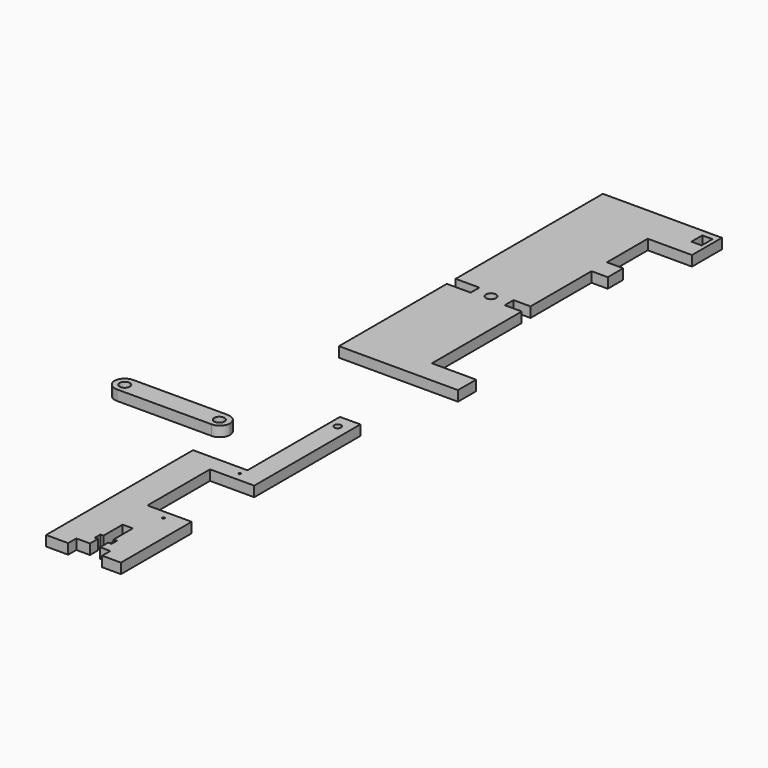
from build123d import *

# Parameters (mm, degrees)
F0_W        = 34
F0_H        = 6
F1_DEPTH    = 3
F2_T1_DEPTH = 18.5
F3_T1_DEPTH = 18.5
F4_R        = 1.5
F5_DEPTH    = 25.8
F6_W        = 35
F6_H        = 97
F7_DEPTH    = 3
F9_DEPTH    = 65
F10_W       = 13
F10_H       = 58.6508959532
F11_DEPTH   = 25
F12_W       = 5
F12_H       = 3.23662889
F12_W_2     = 7
F12_H_2     = 3.2004637718
F13_DEPTH   = 35.3
F14_R       = 1.5
F15_DEPTH   = 25
F16_W       = 8.2240308821
F16_H       = 5.6709373705
F16_W_2     = 3
F16_H_2     = 4
F17_DEPTH   = 25
F18_W       = 22
F18_H       = 88
F19_DEPTH   = 3
F20_W       = 16
F20_H       = 34
F21_DEPTH   = 14.5
F22_W       = 13
F22_H       = 23
F23_DEPTH   = 25
F24_W       = 10
F24_H       = 3
F25_DEPTH   = 25
F26_W       = 3
F26_H       = 12
F27_DEPTH   = 25
F29_DEPTH   = 25
F30_R       = 1
F30_R_2     = 0.35
F31_DEPTH   = 25


# Not quite as in the source:
# - a fillet or chamfer that OpenCascade refuses, or shapes differently, is made with other operations: its cross-section is extruded or revolved along the edge and cut away or added


with BuildPart() as f1:
    # F0 (on Top) → F1 (new body)
    with BuildSketch(Plane.XY):
        with Locations((-28.7276850939, -1.7022728249)):
            Rectangle(F0_W, F0_H)
    extrude(amount=F1_DEPTH)

    # F2: fillet of radius 3.1 on 2 edges, made by hand

    # F2_s2 → F2_t1 (cut)
    with BuildSketch(Plane.XY.offset(-7.75)):
        with BuildLine():
            ThreePointArc((-14.8276850939, -4.7022728249), (-12.6356540722, -3.7943038466), (-11.7276850939, -1.6022728249))
            Line((-11.7276850939, -1.6022728249), (-11.7276850939, -4.7022728249))
            Line((-11.7276850939, -4.7022728249), (-14.8276850939, -4.7022728249))
        make_face()
        with BuildLine():
            ThreePointArc((-14.8276850939, 1.2977271751), (-12.6356540722, 0.3897581967), (-11.7276850939, -1.8022728249))
            Line((-11.7276850939, -1.8022728249), (-11.7276850939, 1.2977271751))
            Line((-11.7276850939, 1.2977271751), (-14.8276850939, 1.2977271751))
        make_face()
    extrude(amount=F2_T1_DEPTH, mode=Mode.SUBTRACT)

    # F3: fillet of radius 3.1 on 2 edges, made by hand

    # F3_s2 → F3_t1 (cut)
    with BuildSketch(Plane.XY.offset(-7.75)):
        with BuildLine():
            ThreePointArc((-45.7276850939, -1.6022728249), (-44.8197161156, -3.7943038466), (-42.6276850939, -4.7022728249))
            Line((-42.6276850939, -4.7022728249), (-45.7276850939, -4.7022728249))
            Line((-45.7276850939, -4.7022728249), (-45.7276850939, -1.6022728249))
        make_face()
        with BuildLine():
            ThreePointArc((-42.6276850939, 1.2977271751), (-44.8197161156, 0.3897581967), (-45.7276850939, -1.8022728249))
            Line((-45.7276850939, -1.8022728249), (-45.7276850939, 1.2977271751))
            Line((-45.7276850939, 1.2977271751), (-42.6276850939, 1.2977271751))
        make_face()
    extrude(amount=F3_T1_DEPTH, mode=Mode.SUBTRACT)

    # F4 (on face) → F5 (cut)
    with BuildSketch(Plane(origin=(0, 0, 0), x_dir=(1, 0, 0), z_dir=(0, 0, -1))):
        with Locations((-42.6276850939, 1.8022728249)):
            Circle(F4_R)
        with Locations((-14.8276850939, 1.8022728249)):
            Circle(F4_R)
    extrude(amount=-F5_DEPTH, mode=Mode.SUBTRACT)


with BuildPart() as f7:
    # F6 (on Top) → F7 (new body)
    with BuildSketch(Plane.XY):
        with Locations((1.2659030035, 92.4109403007)):
            Rectangle(F6_W, F6_H)
    extrude(amount=F7_DEPTH)

    # F8 (on face) → F9 (cut)
    with BuildSketch(Plane.XY.offset(3)):
        Polygon((18.7659030035, 114.9109403007), (18.7659030035, 129.9109403007), (14.4255761913, 129.9109403007), (5.7659030035, 129.9109403007), (5.7659030035, 114.9109403007), align=None)
    extrude(amount=-F9_DEPTH, mode=Mode.SUBTRACT)

    # F10 (on face) → F11 (cut)
    with BuildSketch(Plane.XY.offset(3)):
        with Locations((12.2659030035, 79.9145549536)):
            Rectangle(F10_W, F10_H)
    extrude(amount=-F11_DEPTH, mode=Mode.SUBTRACT)

    # F12 (on face) → F13 (cut)
    with BuildSketch(Plane.XY.offset(3)):
        with Locations((3.2659030035, 85.207421422)):
            Rectangle(F12_W, F12_H)
        with Locations((-12.7340969965, 85.1893388629)):
            Rectangle(F12_W_2, F12_H_2)
    extrude(amount=-F13_DEPTH, mode=Mode.SUBTRACT)

    # F14 (on face) → F15 (cut)
    with BuildSketch(Plane.XY.offset(3)):
        with Locations((-4.4696778059, 85.0904509425)):
            Circle(F14_R)
    extrude(amount=-F15_DEPTH, mode=Mode.SUBTRACT)

    # F16 (on face) → F17 (cut)
    with BuildSketch(Plane.XY.offset(3)):
        with Locations((14.6538875625, 112.0754716154)):
            Rectangle(F16_W, F16_H)
        with Locations((16.0067553967, 137.0250095129)):
            Rectangle(F16_W_2, F16_H_2)
    extrude(amount=-F17_DEPTH, mode=Mode.SUBTRACT)


with BuildPart() as f19:
    # F18 (on Top) → F19 (new body)
    with BuildSketch(Plane.XY):
        with Locations((0.9128389647, -27.3907984654)):
            Rectangle(F18_W, F18_H)
    extrude(amount=F19_DEPTH)

    # F20 (on face) → F21 (cut)
    with BuildSketch(Plane.XY.offset(3)):
        with Locations((-2.0871610353, -0.3907984654)):
            Rectangle(F20_W, F20_H)
    extrude(amount=-F21_DEPTH, mode=Mode.SUBTRACT)

    # F22 (on face) → F23 (cut)
    with BuildSketch(Plane.XY.offset(3)):
        with Locations((5.4128389647, -33.8907984654)):
            Rectangle(F22_W, F22_H)
    extrude(amount=-F23_DEPTH, mode=Mode.SUBTRACT)

    # F24 (on face) → F25 (cut)
    with BuildSketch(Plane.XY.offset(3)):
        with Locations((1.4128389647, -69.8907984654)):
            Rectangle(F24_W, F24_H)
    extrude(amount=-F25_DEPTH, mode=Mode.SUBTRACT)

    # F26 (on face) → F27 (cut)
    with BuildSketch(Plane.XY.offset(3)):
        with Locations((1.9128389647, -62.3907984654)):
            Rectangle(F26_W, F26_H)
    extrude(amount=-F27_DEPTH, mode=Mode.SUBTRACT)

    # F28 (on face) → F29 (cut)
    with BuildSketch(Plane.XY.offset(3)):
        Polygon((-0.4876649764, -63.4444471002), (-0.4876649764, -65.4444471002), (0.4128389647, -65.4444471002), (4.4208336622, -65.4444471002), (4.4208336622, -63.4444471002), align=None)
    extrude(amount=-F29_DEPTH, mode=Mode.SUBTRACT)

    # F30 (on face) → F31 (cut)
    with BuildSketch(Plane.XY.offset(3)):
        with Locations((8.4350015968, 12.605776079)):
            Circle(F30_R)
        with Locations((5.5628389647, -19.772477448)):
            Circle(F30_R_2)
        with Locations((5.6899152696, -47.9949377477)):
            Circle(F30_R_2)
    extrude(amount=-F31_DEPTH, mode=Mode.SUBTRACT)


solid = Compound([f1.part, f7.part, f19.part])
